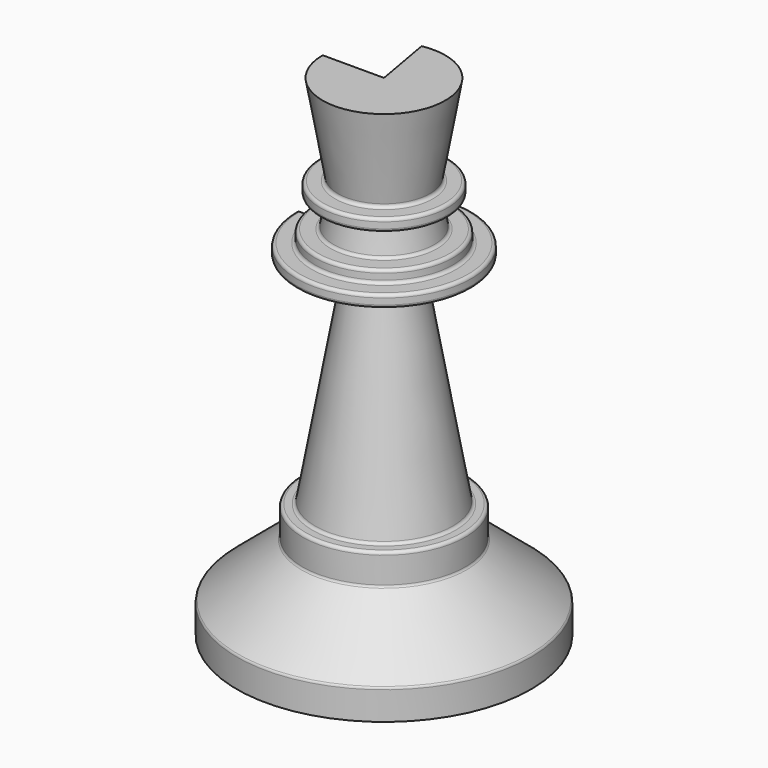
from build123d import *

# Parameters (mm, degrees)
F1_ANGLE = 280


# Not quite as in the source:
# - a feature of the source that left no trace in its solid (it failed there, or was rolled back) is left out


with BuildPart() as f1:
    # F0 (on Front) → F1 (revolve)
    with BuildSketch(Plane.XZ):
        with BuildLine():
            Line((-15.24, 0), (0, 0))
            Line((0, 0), (0, 50.8))
            Line((0, 50.8), (-6.35, 50.8))
            Line((-6.35, 50.8), (-4.7617064118, 41.792339449))
            ThreePointArc((-4.7617064118, 41.792339449), (-4.8311637627, 41.5331210865), (-5.0743828734, 41.4197061526))
            Line((-5.0743828734, 41.4197061526), (-6.2835011077, 41.4197061526))
            ThreePointArc((-6.2835011077, 41.4197061526), (-6.5080075107, 41.3267125556), (-6.6010011077, 41.1022061526))
            Line((-6.6010011077, 41.1022061526), (-6.6010011077, 40.4672061526))
            ThreePointArc((-6.6010011077, 40.4672061526), (-6.5080075107, 40.2426997495), (-6.2835011077, 40.1497061526))
            Line((-6.2835011077, 40.1497061526), (-5.0743828734, 40.1497061526))
            ThreePointArc((-5.0743828734, 40.1497061526), (-4.8311637627, 40.0362912186), (-4.7617064118, 39.7770728561))
            Line((-4.7617064118, 39.7770728561), (-5.2010717431, 37.2853082403))
            ThreePointArc((-5.2010717431, 37.2853082403), (-5.3096631386, 37.0972224261), (-5.5137482047, 37.0229415367))
            Line((-5.5137482047, 37.0229415367), (-6.8348340718, 37.0229415367))
            ThreePointArc((-6.8348340718, 37.0229415367), (-7.0593404748, 36.9299479398), (-7.1523340718, 36.7054415367))
            Line((-7.1523340718, 36.7054415367), (-7.1523340718, 36.0704415367))
            ThreePointArc((-7.1523340718, 36.0704415367), (-7.2453276688, 35.8459351337), (-7.4698340718, 35.7529415367))
            Line((-7.4698340718, 35.7529415367), (-8.7398340718, 35.7529415367))
            ThreePointArc((-8.7398340718, 35.7529415367), (-8.9643404748, 35.6599479398), (-9.0573340718, 35.4354415367))
            Line((-9.0573340718, 35.4354415367), (-9.0573340718, 34.8004415367))
            ThreePointArc((-9.0573340718, 34.8004415367), (-8.9643404748, 34.5759351337), (-8.7398340718, 34.4829415367))
            Line((-8.7398340718, 34.4829415367), (-3.5686493249, 34.4829415367))
            ThreePointArc((-3.5686493249, 34.4829415367), (-3.3254302142, 34.3695266028), (-3.2559728633, 34.1103082403))
            Line((-3.2559728633, 34.1103082403), (-7.113602572, 12.2326030065))
            ThreePointArc((-7.113602572, 12.2326030065), (-7.2221939675, 12.0445171922), (-7.4262790336, 11.9702363029))
            Line((-7.4262790336, 11.9702363029), (-8.1123649007, 11.9702363029))
            ThreePointArc((-8.1123649007, 11.9702363029), (-8.3368713037, 11.8772427059), (-8.4298649007, 11.6527363029))
            Line((-8.4298649007, 11.6527363029), (-8.4298649007, 8.9432889844))
            ThreePointArc((-8.4298649007, 8.9432889844), (-8.4596121783, 8.8091076862), (-8.5432798346, 8.7000698737))
            Line((-8.5432798346, 8.7000698737), (-15.1265850661, 3.176020882))
            ThreePointArc((-15.1265850661, 3.176020882), (-15.2102527224, 3.0669830694), (-15.24, 2.9328017713))
            Line((-15.24, 2.9328017713), (-15.24, 0))
        make_face()
    revolve(axis=Axis((0, 0, 25.4), (0, 0, 1)), revolution_arc=F1_ANGLE)


solid = f1.part
